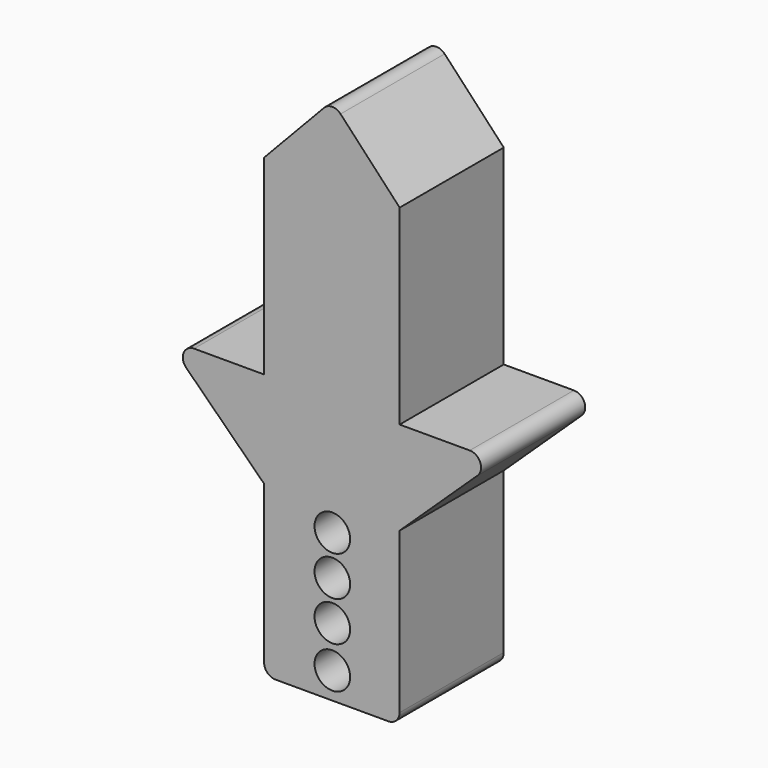
from build123d import *

# Parameters (mm, degrees)
F1_DEPTH = 25.4
F2_R     = 3.4757285613
F3_DEPTH = 25.401
F6_R     = 2.2115163873


# Not quite as in the source:
# - the program builds the solid bodies; features that only make, move or delete a surface that nothing else refers to are left out


with BuildPart() as f1:
    # F0 (on Front) → F1 (new body)
    with BuildSketch(Plane.XZ):
        Polygon((-13.319584541, 37.2763350606), (-13.319584541, 0), (-32.3739908636, 0), (-13.319584541, -18.7769141048), (-13.319584541, -51.7058856785), (13.1345912814, -51.7058856785), (13.1345912814, -18.221931532), (32.3739871383, 0), (13.1345912814, 0), (13.1345912814, 37.2763350606), (0, 51.3358972967), align=None)
    extrude(amount=F1_DEPTH)

    # F2 (on Front) → F3 (cut, through all)
    with BuildSketch(Plane.XZ):
        with Locations((0, -22.8467863053)):
            Circle(F2_R)
        with Locations((0, -30.6165441871)):
            Circle(F2_R)
        with Locations((0, -38.3863002062)):
            Circle(F2_R)
        with Locations((0, -46.5260483325)):
            Circle(F2_R)
    extrude(amount=F3_DEPTH, mode=Mode.SUBTRACT)

    # F6
    f6_edges = [f1.edges().sort_by_distance(p)[0] for p in [
        (-32.373991, -12.7, 0),
        (32.373987, -12.7, 0),
        (-13.319585, -12.7, -51.705886),
        (13.134591, -12.7, -51.705886),
        (0, -12.7, 51.335897),
    ]]
    fillet(f6_edges, radius=F6_R)


solid = f1.part
